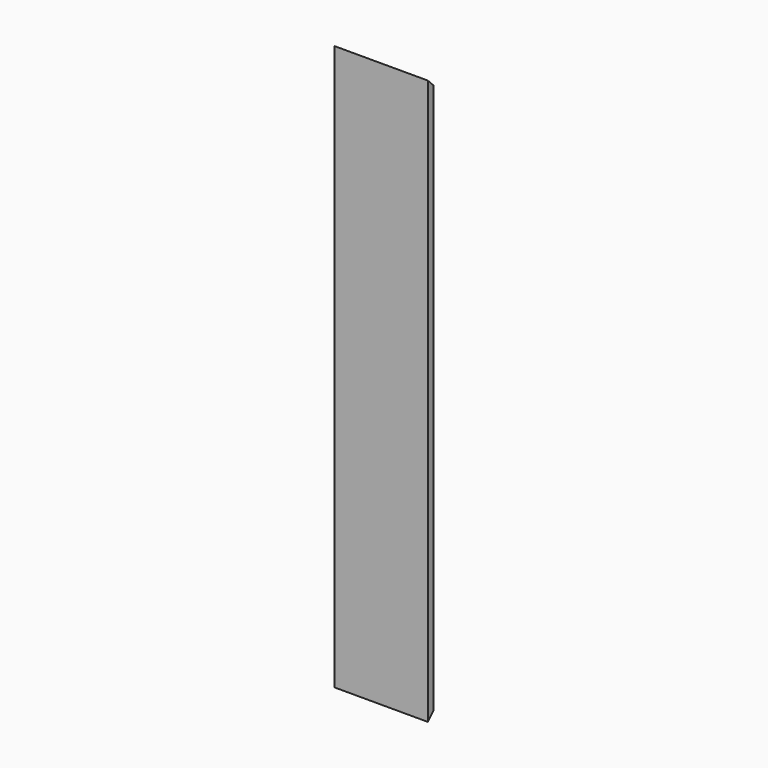
from build123d import *

# Parameters (mm, degrees)
F0_W     = 254
F0_H     = 19.05
F1_DEPTH = 768.35
F2_SIZE2 = 19.04999
F2_SIZE  = 19.04999


# Not quite as in the source:
# - a fillet or chamfer is up to 0.001 mm smaller than in the source, because OpenCascade refuses the exact size


with BuildPart() as f1:
    # F0 (on Top) → F1 (new body, symmetric)
    with BuildSketch(Plane.XY):
        Rectangle(F0_W, F0_H)
    extrude(amount=F1_DEPTH, both=True)

    # F2 (size 19.05 and 19.05 in the source; OpenCascade refuses exactly that, so slightly less here)
    f2_edges = [f1.edges().sort_by_distance(p)[0] for p in [
        (0, 9.525, 768.35),
        (0, 9.525, -768.35),
    ]]
    chamfer(f2_edges, length=F2_SIZE, length2=F2_SIZE2)


solid = f1.part
